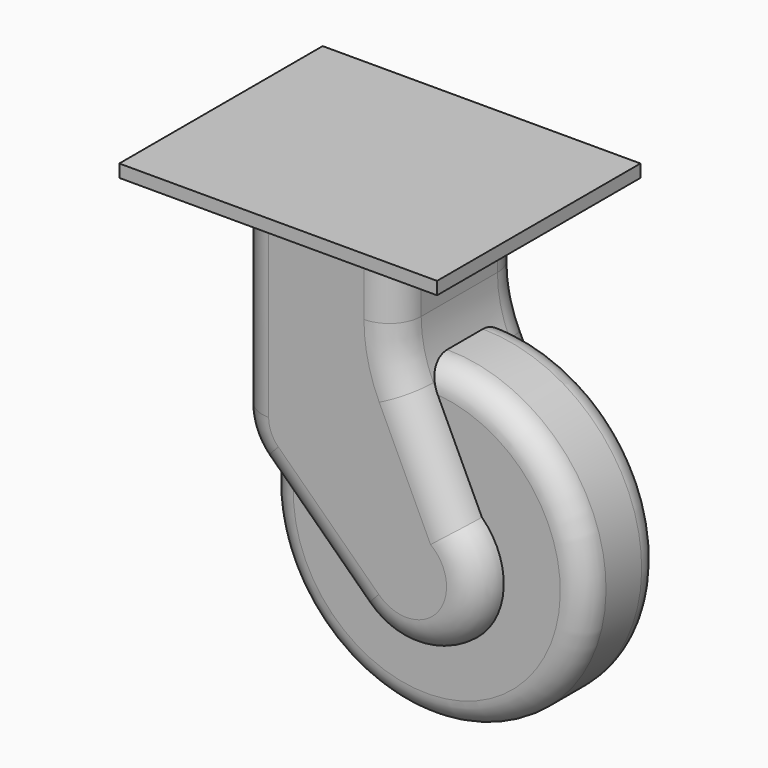
from build123d import *

# Parameters (mm, degrees)
F0_W     = 50
F0_H     = 40
F1_DEPTH = 2
F3_DEPTH = 12.5
F4_R     = 25
F5_DEPTH = 7.5
F6_R     = 4
F7_R     = 4.99999


# Not quite as in the source:
# - a fillet or chamfer is up to 0.001 mm smaller than in the source, because OpenCascade refuses the exact size


with BuildPart() as f1:
    # F0 (on Top) → F1 (new body)
    with BuildSketch(Plane.XY):
        Rectangle(F0_W, F0_H)
    extrude(amount=F1_DEPTH)

    # F2 (on Front) → F3 (join, symmetric)
    with BuildSketch(Plane.XZ):
        with BuildLine():
            Line((12.5, 0), (-12.5, 0))
            Line((-12.5, 0), (-12.5, -30.5279912201))
            ThreePointArc((-12.5, -30.5279912201), (-11.7069556163, -34.43080665), (-9.4536063441, -37.7146009084))
            Line((-9.4536063441, -37.7146009084), (6.3529476633, -53.0086768346))
            ThreePointArc((6.3529476633, -53.0086768346), (22.3177107814, -52.745608492), (22.0546424389, -36.7808453739))
            Line((22.0546424389, -36.7808453739), (14.4186308033, -20.6281161927))
            ThreePointArc((14.4186308033, -20.6281161927), (12.9855517125, -16.4605806119), (12.5, -12.0803628053))
            Line((12.5, -12.0803628053), (12.5, 0))
        make_face()
    extrude(amount=F3_DEPTH, both=True)

    # F4 (on Front) → F5 (join, symmetric)
    with BuildSketch(Plane.XZ):
        with Locations((13.390565291, -43)):
            Circle(F4_R)
    extrude(amount=F5_DEPTH, both=True)

    # F6
    f6_edges = [f1.edges().sort_by_distance(p)[0] for p in [
        (28.500684, -7.5, -62.916935),
        (28.500684, 7.5, -62.916935),
    ]]
    fillet(f6_edges, radius=F6_R)

    # F7 (radius 5 in the source; OpenCascade refuses exactly that, so slightly less here)
    f7_edges = [f1.edges().sort_by_distance(p)[0] for p in [
        (12.5, -12.5, -6.040181),
        (-12.5, -12.5, -15.263996),
        (-12.5, 12.5, -15.263996),
        (12.5, 12.5, -6.040181),
    ]]
    fillet(f7_edges, radius=F7_R)


solid = f1.part
